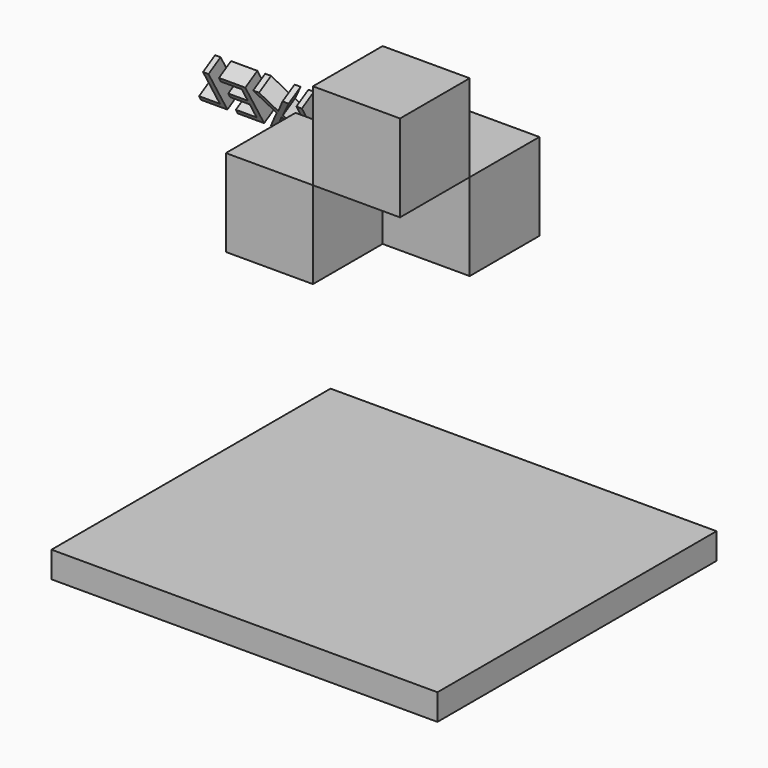
from build123d import *

# Parameters (mm, degrees)
F0_W         = 10
F0_H         = 10
F1_DEPTH     = 10
F2_W         = 10
F2_H         = 10
F3_DEPTH     = 10
F4_W         = 10
F4_H         = 10
F5_DEPTH     = 10
F7_TEXT_SIZE = 7.5929292103
F8_DEPTH     = 2
F9_ANGLE     = 30
F12_W        = 44.3192766979
F12_H        = 40.0548800826
F13_DEPTH    = 3


# Not quite as in the source:
# - Text() gives the source's letters only with a copy of the font that has no kerning and outlines rounded to 1/6400 em; it was checked with that copy


with BuildPart() as f1:
    # F0 (on Front) → F1 (new body)
    with BuildSketch(Plane.XZ):
        Rectangle(F0_W, F0_H)
    extrude(amount=F1_DEPTH)


with BuildPart() as f3:
    # F2 (on face) → F3 (new body)
    with BuildSketch(Plane(origin=(-5, 0, 0), x_dir=(0, -1, 0), z_dir=(-1, 0, 0))):
        with Locations((15, 10)):
            Rectangle(F2_W, F2_H)
    extrude(amount=-F3_DEPTH)


with BuildPart() as f5:
    # F4 (on face) → F5 (new body)
    with BuildSketch(Plane(origin=(-5, 0, 0), x_dir=(0, -1, 0), z_dir=(-1, 0, 0))):
        with Locations((15, 0)):
            Rectangle(F4_W, F4_H)
    extrude(amount=F5_DEPTH)


with BuildPart() as f8:
    # F7 (on offset) → F8 (new body)
    with BuildSketch(Plane(origin=(0, -5, 0), x_dir=(-1, 0, 0), z_dir=(0, 1, 0))):
        with Locations((8.0287111923, -4.2550959624)):
            Text('TRIXEL', F7_TEXT_SIZE, font='Open Sans', text_align=(TextAlign.LEFT, TextAlign.BOTTOM))
    extrude(amount=F8_DEPTH)


with BuildPart() as f8_1:
    # F9: moved
    add(f8.part.rotate(Axis((-10, -10, -5), (1, 0, 0)), F9_ANGLE))


with BuildPart() as f8_2:
    # F10: moved
    add(f8_1.part.moved(Location((0, 3, 0))))


with BuildPart() as f13:
    # F12 (on offset) → F13 (new body)
    with BuildSketch(Plane(origin=(0, 0, -35), x_dir=(1, 0, 0), z_dir=(0, 0, -1))):
        with Locations((-4.9361721613, 9.8794102669)):
            Rectangle(F12_W, F12_H)
    extrude(amount=F13_DEPTH)


solid = Compound([f1.part, f3.part, f5.part, f8_2.part, f13.part])
